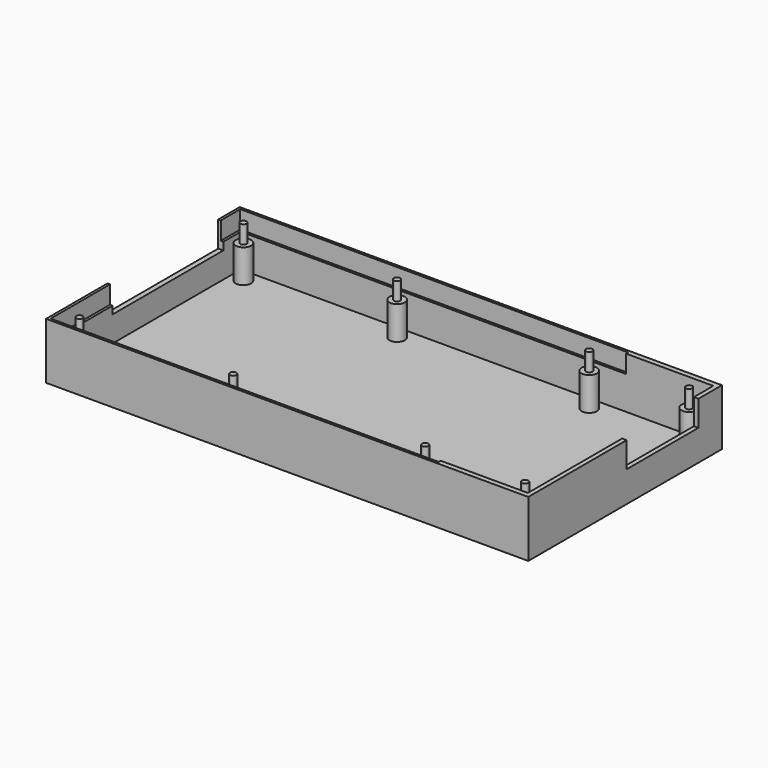
from build123d import *

# Parameters (mm, degrees)
F0_W     = 1
F0_H     = 54
F0_W_2   = 1.75
F0_H_2   = 35
F0_R     = 3
F0_R_2   = 1.25
F1_DEPTH = 2
F2_DEPTH = 20
F3_DEPTH = 13
F4_DEPTH = 10
F5_DEPTH = 20
F6_DEPTH = 13


# Not quite as in the source:
# - a feature names something its author has since deleted; it is built from what else it names


with BuildPart() as f1:
    # F0 (on Top) → F1 (new body)
    with BuildSketch(Plane.XY):
        Polygon((10.25, 0), (-142.25, 0), (-142.25, -10.5), (-141.25, -10.5), (-141.25, -1), (10.25, -1), align=None)
        Polygon((46, 0), (10.25, 0), (10.25, -1), (10.25, -2), (44.25, -2), (44.25, -11.5), (46, -11.5), align=None)
        with Locations((-141.75, -37.5)):
            Rectangle(F0_W, F0_H)
        Polygon((10.25, -2), (10.25, -1), (-141.25, -1), (-141.25, -10.5), (-140.25, -10.5), (-140.25, -2), align=None)
        Polygon((-141.25, -64.5), (-142.25, -64.5), (-142.25, -94.5), (10.25, -94.5), (10.25, -93.5), (-141.25, -93.5), align=None)
        with Locations((-140.75, -37.5)):
            Rectangle(F0_W, F0_H)
        with Locations((45.125, -29)):
            Rectangle(F0_W_2, F0_H_2)
        Polygon((44.25, -2), (10.25, -2), (-140.25, -2), (-140.25, -10.5), (-140.25, -64.5), (-140.25, -92.5), (10.25, -92.5), (44.25, -92.5), (44.25, -46.5), (44.25, -11.5), align=None)
        with Locations((-135, -87.25)):
            Circle(F0_R, mode=Mode.SUBTRACT)
        with Locations((-75, -87.25)):
            Circle(F0_R, mode=Mode.SUBTRACT)
        with Locations((0, -87.25)):
            Circle(F0_R, mode=Mode.SUBTRACT)
        with Locations((39, -87.25)):
            Circle(F0_R, mode=Mode.SUBTRACT)
        with Locations((-135, -7.25)):
            Circle(F0_R, mode=Mode.SUBTRACT)
        with Locations((-75, -7.25)):
            Circle(F0_R, mode=Mode.SUBTRACT)
        with Locations((0, -7.25)):
            Circle(F0_R, mode=Mode.SUBTRACT)
        with Locations((39, -7.25)):
            Circle(F0_R, mode=Mode.SUBTRACT)
        Polygon((-140.25, -64.5), (-141.25, -64.5), (-141.25, -93.5), (10.25, -93.5), (10.25, -92.5), (-140.25, -92.5), align=None)
        Polygon((46, -94.5), (46, -46.5), (44.25, -46.5), (44.25, -92.5), (10.25, -92.5), (10.25, -93.5), (10.25, -94.5), align=None)
        with Locations((-135, -87.25)):
            Circle(F0_R)
        with Locations((-135, -87.25)):
            Circle(F0_R_2, mode=Mode.SUBTRACT)
        with Locations((-135, -7.25)):
            Circle(F0_R)
        with Locations((-135, -7.25)):
            Circle(F0_R_2, mode=Mode.SUBTRACT)
        with Locations((-75, -87.25)):
            Circle(F0_R)
        with Locations((-75, -87.25)):
            Circle(F0_R_2, mode=Mode.SUBTRACT)
        with Locations((-75, -7.25)):
            Circle(F0_R)
        with Locations((-75, -7.25)):
            Circle(F0_R_2, mode=Mode.SUBTRACT)
        with Locations((0, -7.25)):
            Circle(F0_R)
        with Locations((0, -7.25)):
            Circle(F0_R_2, mode=Mode.SUBTRACT)
        with Locations((0, -87.25)):
            Circle(F0_R)
        with Locations((0, -87.25)):
            Circle(F0_R_2, mode=Mode.SUBTRACT)
        with Locations((39, -87.25)):
            Circle(F0_R)
        with Locations((39, -87.25)):
            Circle(F0_R_2, mode=Mode.SUBTRACT)
        with Locations((39, -7.25)):
            Circle(F0_R)
        with Locations((39, -7.25)):
            Circle(F0_R_2, mode=Mode.SUBTRACT)
        with Locations((-135, -87.25)):
            Circle(F0_R_2)
        with Locations((-75, -87.25)):
            Circle(F0_R_2)
        with Locations((0, -87.25)):
            Circle(F0_R_2)
        with Locations((39, -87.25)):
            Circle(F0_R_2)
        with Locations((-135, -7.25)):
            Circle(F0_R_2)
        with Locations((-75, -7.25)):
            Circle(F0_R_2)
        with Locations((0, -7.25)):
            Circle(F0_R_2)
        with Locations((39, -7.25)):
            Circle(F0_R_2)
    extrude(amount=-F1_DEPTH)

    # F0 (on Top) → F2 (join)
    with BuildSketch(Plane.XY):
        Polygon((10.25, 0), (-142.25, 0), (-142.25, -10.5), (-141.25, -10.5), (-141.25, -1), (10.25, -1), align=None)
        Polygon((46, 0), (10.25, 0), (10.25, -1), (10.25, -2), (44.25, -2), (44.25, -11.5), (46, -11.5), align=None)
        Polygon((46, -94.5), (46, -46.5), (44.25, -46.5), (44.25, -92.5), (10.25, -92.5), (10.25, -93.5), (10.25, -94.5), align=None)
        Polygon((-141.25, -64.5), (-142.25, -64.5), (-142.25, -94.5), (10.25, -94.5), (10.25, -93.5), (-141.25, -93.5), align=None)
    extrude(amount=F2_DEPTH)

    # F0 (on Top) → F3 (join)
    with BuildSketch(Plane.XY):
        Polygon((10.25, -2), (10.25, -1), (-141.25, -1), (-141.25, -10.5), (-140.25, -10.5), (-140.25, -2), align=None)
        Polygon((-140.25, -64.5), (-141.25, -64.5), (-141.25, -93.5), (10.25, -93.5), (10.25, -92.5), (-140.25, -92.5), align=None)
    extrude(amount=F3_DEPTH)

    # F0 (on Top) → F4 (join)
    with BuildSketch(Plane.XY):
        with Locations((-140.75, -37.5)):
            Rectangle(F0_W, F0_H)
        with Locations((-141.75, -37.5)):
            Rectangle(F0_W, F0_H)
        with Locations((45.125, -29)):
            Rectangle(F0_W_2, F0_H_2)
    extrude(amount=F4_DEPTH)

    # F0 (on Top) → F5 (join)
    with BuildSketch(Plane.XY):
        with Locations((-135, -7.25)):
            Circle(F0_R_2)
        with Locations((-75, -7.25)):
            Circle(F0_R_2)
        with Locations((0, -7.25)):
            Circle(F0_R_2)
        with Locations((39, -7.25)):
            Circle(F0_R_2)
        with Locations((39, -87.25)):
            Circle(F0_R_2)
        with Locations((0, -87.25)):
            Circle(F0_R_2)
        with Locations((-75, -87.25)):
            Circle(F0_R_2)
        with Locations((-135, -87.25)):
            Circle(F0_R_2)
    extrude(amount=F5_DEPTH)

    # F0 (on Top) → F6 (join)
    with BuildSketch(Plane.XY):
        with Locations((-135, -7.25)):
            Circle(F0_R)
        with Locations((-135, -7.25)):
            Circle(F0_R_2, mode=Mode.SUBTRACT)
        with Locations((-75, -7.25)):
            Circle(F0_R)
        with Locations((-75, -7.25)):
            Circle(F0_R_2, mode=Mode.SUBTRACT)
        with Locations((0, -7.25)):
            Circle(F0_R)
        with Locations((0, -7.25)):
            Circle(F0_R_2, mode=Mode.SUBTRACT)
        with Locations((39, -7.25)):
            Circle(F0_R)
        with Locations((39, -7.25)):
            Circle(F0_R_2, mode=Mode.SUBTRACT)
        with Locations((-135, -87.25)):
            Circle(F0_R)
        with Locations((-135, -87.25)):
            Circle(F0_R_2, mode=Mode.SUBTRACT)
        with Locations((-75, -87.25)):
            Circle(F0_R)
        with Locations((-75, -87.25)):
            Circle(F0_R_2, mode=Mode.SUBTRACT)
        with Locations((0, -87.25)):
            Circle(F0_R)
        with Locations((0, -87.25)):
            Circle(F0_R_2, mode=Mode.SUBTRACT)
        with Locations((39, -87.25)):
            Circle(F0_R)
        with Locations((39, -87.25)):
            Circle(F0_R_2, mode=Mode.SUBTRACT)
    extrude(amount=F6_DEPTH)


solid = f1.part
